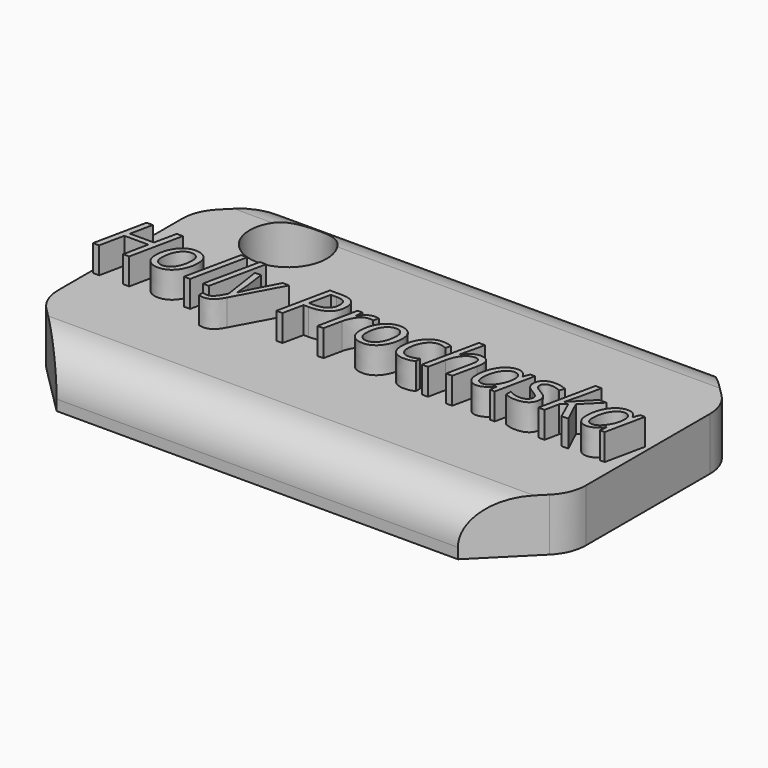
from build123d import *

# Parameters (mm, degrees)
F0_W         = 63.5
F0_H         = 38.1
F1_DEPTH     = 6.35
F2_TEXT_SIZE = 8.9285321968
F3_DEPTH     = 3.175
F4_SIZE      = 7.62
F5_R         = 5.08
F6_R         = 5.08
F7_R         = 4.6379603357
F8_DEPTH     = 25.4


# Not quite as in the source:
# - Text() gives the source's letters only with a copy of the font that has no kerning and outlines rounded to 1/6400 em; it was checked with that copy


with BuildPart() as f1:
    # F0 (on Top) → F1 (new body)
    with BuildSketch(Plane.XY):
        with Locations((31.75, 19.05)):
            Rectangle(F0_W, F0_H)
    extrude(amount=F1_DEPTH)

    # F2 (on face) → F3 (join)
    with BuildSketch(Plane.XY.offset(6.35)):
        with Locations((0, 14.526747266)):
            Text('Holly Prochaska', F2_TEXT_SIZE, font='Open Sans', font_style=FontStyle.ITALIC, text_align=(TextAlign.LEFT, TextAlign.BOTTOM))
    extrude(amount=F3_DEPTH)

    # F4
    f4_edges = [f1.edges().sort_by_distance(p)[0] for p in [
        (63.5, 38.1, 3.175),
        (63.5, 0, 3.175),
        (0, 38.1, 3.175),
        (0, 0, 3.175),
    ]]
    chamfer(f4_edges, length=F4_SIZE)

    # F5
    f5_edges = [f1.edges().sort_by_distance(p)[0] for p in [
        (31.75, 38.1, 6.35),
        (31.75, 0, 6.35),
    ]]
    fillet(f5_edges, radius=F5_R)

    # F6
    f6_edges = [f1.edges().sort_by_distance(p)[0] for p in [
        (0, 30.48, 3.175),
        (63.5, 30.48, 3.175),
        (63.5, 7.62, 3.175),
        (0, 7.62, 3.175),
    ]]
    fillet(f6_edges, radius=F6_R)

    # F7 (on face) → F8 (cut)
    with BuildSketch(Plane.XY.offset(6.35)):
        with Locations((11.0565179676, 30.5154746546)):
            Circle(F7_R)
    extrude(amount=-F8_DEPTH, mode=Mode.SUBTRACT)


solid = f1.part
